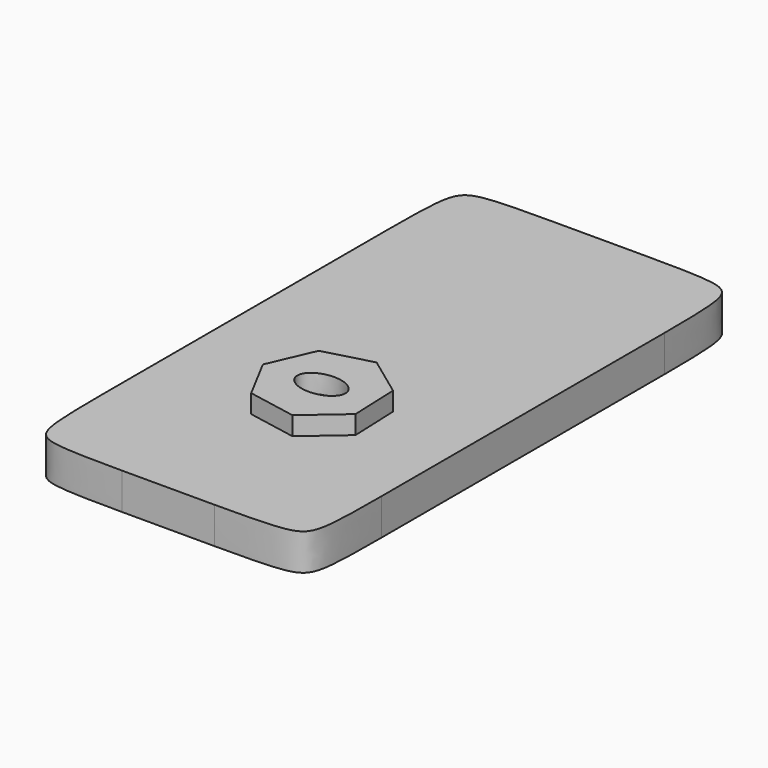
from build123d import *

# Parameters (mm, degrees)
F0_W        = 38.1
F0_H        = 5
F1_DEPTH    = 73.914
F2_T1_DEPTH = 68.5
F5_DEPTH    = 2.54


# Not quite as in the source:
# - a fillet or chamfer that OpenCascade refuses, or shapes differently, is made with other operations: its cross-section is extruded or revolved along the edge and cut away or added


with BuildPart() as f1:
    # F0 (on Front) → F1 (new body)
    with BuildSketch(Plane.XZ):
        with Locations((19.05, 2.5)):
            Rectangle(F0_W, F0_H)
    extrude(amount=F1_DEPTH)

    # F2: fillet of radius 12.7 on 4 edges, made by hand

    # F2_s2 → F2_t1 (cut)
    with BuildSketch(Plane.XY.offset(-31.75)):
        with BuildLine():
            add(Edge.make_bspline(
                [(38.1, -61.214), (38.1, -73.914), (25.4, -73.914)],
                knots=[0, 0, 0, 1, 1, 1], degree=2, weights=[1, 4, 1]))
            Line((25.4, -73.914), (38.1, -73.914))
            Line((38.1, -73.914), (38.1, -61.214))
        make_face()
        with BuildLine():
            add(Edge.make_bspline(
                [(0, -12.7), (0, 0), (12.7, 0)],
                knots=[0, 0, 0, 1, 1, 1], degree=2, weights=[1, 4, 1]))
            Line((12.7, 0), (0, 0))
            Line((0, 0), (0, -12.7))
        make_face()
        with BuildLine():
            add(Edge.make_bspline(
                [(38.1, -12.7), (38.1, 0), (25.4, 0)],
                knots=[0, 0, 0, 1, 1, 1], degree=2, weights=[1, 4, 1]))
            Line((25.4, 0), (38.1, 0))
            Line((38.1, 0), (38.1, -12.7))
        make_face()
        with BuildLine():
            add(Edge.make_bspline(
                [(0, -61.214), (0, -73.914), (12.7, -73.914)],
                knots=[0, 0, 0, 1, 1, 1], degree=2, weights=[1, 4, 1]))
            Line((12.7, -73.914), (0, -73.914))
            Line((0, -73.914), (0, -61.214))
        make_face()
    extrude(amount=F2_T1_DEPTH, mode=Mode.SUBTRACT)


with BuildPart() as f5:
    # F4 (on face) → F5 (new body)
    with BuildSketch(Plane.XY.offset(5)):
        Polygon((21.9590889072, -56.2922066174), (27.0755512858, -51.8682369866), (26.8068146657, -45.1097256716), (21.3552432029, -41.1059695411), (14.8259814009, -42.8718786231), (12.1356965691, -49.0776873608), (15.3102280577, -55.0502951994), align=None)
        with BuildLine():
            add(Edge.make_bspline(
                [(23.230788256, -48.768), (23.230788256, -44.9860916248), (18.2707353197, -46.8770458124), (13.3106823833, -48.768), (18.2707353197, -50.6589541876), (23.230788256, -52.5499083752), (23.230788256, -48.768)],
                knots=[0, 0, 0, 2.0943951024, 2.0943951024, 4.1887902048, 4.1887902048, 6.2831853072, 6.2831853072, 6.2831853072], degree=2, weights=[1, 0.5, 1, 0.5, 1, 0.5, 1]))
        make_face(mode=Mode.SUBTRACT)
    extrude(amount=F5_DEPTH)


solid = Compound([f1.part, f5.part])
